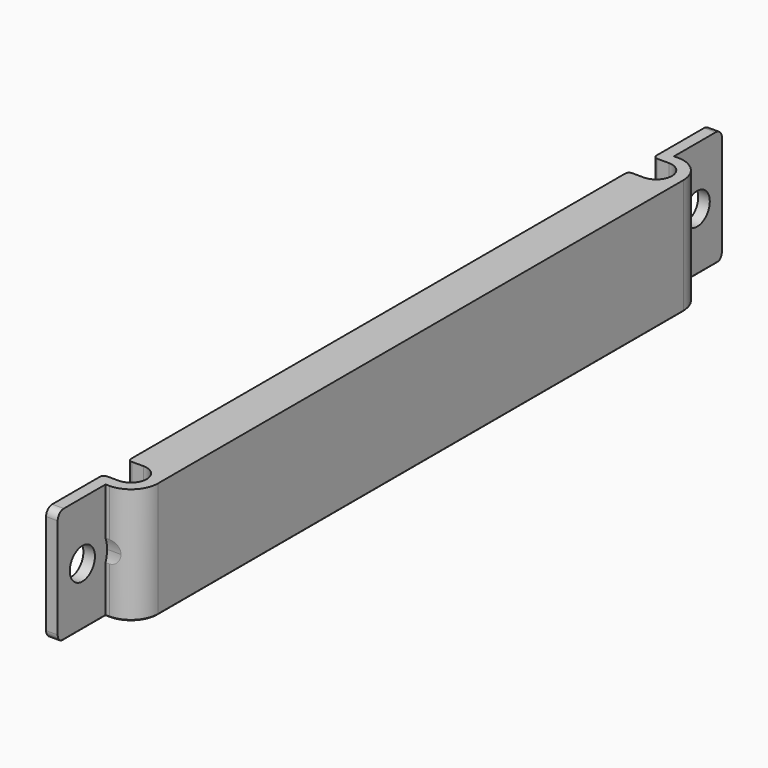
from build123d import *

# Parameters (mm, degrees)
F1_DEPTH     = 15
F2_R         = 1
F3_R         = 4.075
F4_DEPTH     = 3
F3_R_2       = 8
F5_DEPTH     = 8.001
F6_R         = 2
F7_T1_DEPTH  = 16.5429652699
F7_T3_DEPTH  = 3
F7_T5_DEPTH  = 170
F7_T7_DEPTH  = 159.9
F7_T9_DEPTH  = 16.5429652699
F7_T12_ANGLE = 90
F7_T16_DEPTH = 15.2358860169
F7_T21_DEPTH = 1.642920747
F7_T24_ANGLE = 180
F7_T26_ANGLE = 90
F7_T28_ANGLE = 90
F7_T30_ANGLE = 90
F7_T34_DEPTH = 1.642920747
F7_T37_ANGLE = 90
F7_T41_DEPTH = 15.2358860169
F7_T44_ANGLE = 180
F7_T46_ANGLE = 90


# Not quite as in the source:
# - a fillet or chamfer that OpenCascade refuses, or shapes differently, is made with other operations: its cross-section is extruded or revolved along the edge and cut away or added


with BuildPart() as f1:
    # F0 (on Top) → F1 (new body, symmetric)
    with BuildSketch(Plane.XY):
        with BuildLine():
            Line((-4, 89.05), (0, 89.05))
            ThreePointArc((0, 89.05), (4.05, 85), (0, 80.95))
            Line((0, 80.95), (-4, 80.95))
            Line((-4, 80.95), (-4, 0))
            Line((-4, 0), (-4, -80.95))
            Line((-4, -80.95), (0, -80.95))
            ThreePointArc((0, -80.95), (4.05, -85), (0, -89.05))
            Line((0, -89.05), (-4, -89.05))
            Line((-4, -89.05), (-4, -107.5))
            Line((-4, -107.5), (-1, -107.5))
            Line((-1, -107.5), (-1, -92))
            Line((-1, -92), (0, -92))
            ThreePointArc((0, -92), (4.9497474683, -89.9497474683), (7, -85))
            Line((7, -85), (7, 0))
            Line((7, 0), (7, 85))
            ThreePointArc((7, 85), (4.9497474683, 89.9497474683), (0, 92))
            Line((0, 92), (-1, 92))
            Line((-1, 92), (-1, 107.5))
            Line((-1, 107.5), (-4, 107.5))
            Line((-4, 107.5), (-4, 89.05))
        make_face()
    extrude(amount=F1_DEPTH, both=True)

    # F2
    f2_edges = [f1.edges().sort_by_distance(p)[0] for p in [
        (-4, 89.05, 0),
        (-4, 80.95, 0),
        (-4, -89.05, 0),
        (-4, -80.95, 0),
    ]]
    fillet(f2_edges, radius=F2_R)

    # F3 (on face) → F4 (cut, through all)
    with BuildSketch(Plane.YZ.offset(-1)):
        with Locations((99.5, 0)):
            Circle(F3_R)
        with Locations((-99.5, 0)):
            Circle(F3_R)
    extrude(amount=-F4_DEPTH, mode=Mode.SUBTRACT)

    # F3 (on face) → F5 (cut, through all)
    with BuildSketch(Plane.YZ.offset(-1)):
        with Locations((99.5, 0)):
            Circle(F3_R_2)
        with Locations((99.5, 0)):
            Circle(F3_R, mode=Mode.SUBTRACT)
        with BuildLine():
            ThreePointArc((-92, -2.7838821814), (-91.625992126, -1.4142135624), (-91.5, 0))
            ThreePointArc((-91.5, 0), (-91.625992126, 1.4142135624), (-92, 2.7838821814))
            Line((-92, 2.7838821814), (-92, -2.7838821814))
        make_face()
        with BuildLine():
            Line((-92, -2.7838821814), (-92, 2.7838821814))
            ThreePointArc((-92, 2.7838821814), (-100.9142136429, 7.8740078596), (-107.5, -1.636e-07))
            ThreePointArc((-107.5, -1.636e-07), (-100.9142134819, -7.8740078885), (-92, -2.7838821814))
        make_face()
        with Locations((-99.5, 0)):
            Circle(F3_R, mode=Mode.SUBTRACT)
    extrude(amount=F5_DEPTH, mode=Mode.SUBTRACT)

    # F6
    f6_edges = [f1.edges().sort_by_distance(p)[0] for p in [
        (-2.5, 107.5, -15),
        (-2.5, 107.5, 15),
        (-2.5, -107.5, -15),
        (-2.5, -107.5, 15),
    ]]
    fillet(f6_edges, radius=F6_R)

    # F7: chamfer of 0.25 on 22 edges, made by hand

    # F7_s2 → F7_t1 (cut)
    with BuildSketch(Plane.XZ.offset(-106.5929652699)):
        Polygon((-3.75, -15), (-4, -14.75), (-4, -15), align=None)
    extrude(amount=F7_T1_DEPTH, mode=Mode.SUBTRACT)

    # F7_s4 → F7_t3 (cut)
    with BuildSketch(Plane.YZ.offset(-3)):
        Polygon((89.3, -15), (89.05, -14.75), (89.05, -15), align=None)
        Polygon((80.7, -15), (80.95, -14.75), (80.95, -15), align=None)
        Polygon((-80.7, -15), (-80.95, -14.75), (-80.95, -15), align=None)
        Polygon((-89.3, -15), (-89.05, -14.75), (-89.05, -15), align=None)
    extrude(amount=F7_T3_DEPTH, mode=Mode.SUBTRACT)

    # F7_s6 → F7_t5 (cut)
    with BuildSketch(Plane.XZ.offset(-85)):
        Polygon((6.75, -15), (7, -14.75), (7, -15), align=None)
    extrude(amount=F7_T5_DEPTH, mode=Mode.SUBTRACT)

    # F7_s8 → F7_t7 (cut)
    with BuildSketch(Plane.XZ.offset(-79.95)):
        Polygon((-3.75, -15), (-4, -14.75), (-4, -15), align=None)
    extrude(amount=F7_T7_DEPTH, mode=Mode.SUBTRACT)

    # F7_s10 → F7_t9 (cut)
    with BuildSketch(Plane.XZ.offset(90.05)):
        Polygon((-4, -14.75), (-3.75, -15), (-4, -15), align=None)
    extrude(amount=F7_T9_DEPTH, mode=Mode.SUBTRACT)

    # F7_s11 → F7_t12 (revolve, cut)
    with BuildSketch(Plane.YZ.offset(-3)):
        Polygon((89.3, -15), (89.05, -14.75), (89.05, -15), align=None)
    revolve(axis=Axis((-3, 90.05, -15), (0, 0, -1)), revolution_arc=F7_T12_ANGLE, mode=Mode.SUBTRACT)


with BuildPart() as f7_tool14:
    # F7_s15 → F7_t16 (new body)
    with BuildSketch(Plane.XZ.offset(-91.357079253)):
        Polygon((-1.25, -15), (-1, -14.75), (-1, -15), align=None)
    extrude(amount=-F7_T16_DEPTH)

    split(bisect_by=Plane(origin=(0, 53.375, -53.375), x_dir=(1, 0, 0), z_dir=(0, 0.7071067812, -0.7071067812)), keep=Keep.TOP)


with BuildPart() as f1_1:
    add(f1.part)

    # F7_t13: cut F7_tool14
    add(f7_tool14.part, mode=Mode.SUBTRACT)


with BuildPart() as f7_tool19:
    # F7_s20 → F7_t21 (new body)
    with BuildSketch(Plane.YZ):
        Polygon((91.75, -15), (92, -14.75), (92, -15), align=None)
    extrude(amount=-F7_T21_DEPTH)

    split(bisect_by=Plane(origin=(6.875, 0, -6.875), x_dir=(0, 1, 0), z_dir=(0.7071067812, 0, -0.7071067812)), keep=Keep.TOP)


with BuildPart() as f1_2:
    add(f1_1.part)

    # F7_t18: cut F7_tool19
    add(f7_tool19.part, mode=Mode.SUBTRACT)

    # F7_s23 → F7_t24 (revolve, cut)
    with BuildSketch(Plane.YZ):
        Polygon((89.3, -15), (89.05, -14.75), (89.05, -15), align=None)
    revolve(axis=Axis((0, 85, -15), (0, 0, -1)), revolution_arc=F7_T24_ANGLE, mode=Mode.SUBTRACT)

    # F7_s25 → F7_t26 (revolve, cut)
    with BuildSketch(Plane.XZ.offset(-85)):
        Polygon((6.75, -15), (7, -14.75), (7, -15), align=None)
    revolve(axis=Axis((0, 85, -15), (0, 0, 1)), revolution_arc=F7_T26_ANGLE, mode=Mode.SUBTRACT)

    # F7_s27 → F7_t28 (revolve, cut)
    with BuildSketch(Plane.XZ.offset(-79.95)):
        Polygon((-3.75, -15), (-4, -14.75), (-4, -15), align=None)
    revolve(axis=Axis((-3, 79.95, -15), (0, 0, -1)), revolution_arc=F7_T28_ANGLE, mode=Mode.SUBTRACT)

    # F7_s29 → F7_t30 (revolve, cut)
    with BuildSketch(Plane.YZ):
        Polygon((-91.75, -15), (-92, -14.75), (-92, -15), align=None)
    revolve(axis=Axis((0, -85, -15), (0, 0, 1)), revolution_arc=F7_T30_ANGLE, mode=Mode.SUBTRACT)


with BuildPart() as f7_tool32:
    # F7_s33 → F7_t34 (new body)
    with BuildSketch(Plane.YZ.offset(-1.642920747)):
        Polygon((-91.75, -15), (-92, -14.75), (-92, -15), align=None)
    extrude(amount=F7_T34_DEPTH)

    split(bisect_by=Plane(origin=(6.875, 0, -6.875), x_dir=(0, 1, 0), z_dir=(0.7071067812, 0, -0.7071067812)), keep=Keep.TOP)


with BuildPart() as f1_3:
    add(f1_2.part)

    # F7_t31: cut F7_tool32
    add(f7_tool32.part, mode=Mode.SUBTRACT)

    # F7_s36 → F7_t37 (revolve, cut)
    with BuildSketch(Plane.YZ.offset(-3)):
        Polygon((-80.7, -15), (-80.95, -14.75), (-80.95, -15), align=None)
    revolve(axis=Axis((-3, -79.95, -15), (0, 0, -1)), revolution_arc=F7_T37_ANGLE, mode=Mode.SUBTRACT)


with BuildPart() as f7_tool39:
    # F7_s40 → F7_t41 (new body)
    with BuildSketch(Plane.XZ.offset(106.5929652699)):
        Polygon((-1.25, -15), (-1, -14.75), (-1, -15), align=None)
    extrude(amount=-F7_T41_DEPTH)

    split(bisect_by=Plane(origin=(0, -53.375, -53.375), x_dir=(1, 0, 0), z_dir=(0, -0.7071067812, -0.7071067812)), keep=Keep.TOP)


with BuildPart() as f1_4:
    add(f1_3.part)

    # F7_t38: cut F7_tool39
    add(f7_tool39.part, mode=Mode.SUBTRACT)

    # F7_s43 → F7_t44 (revolve, cut)
    with BuildSketch(Plane.YZ):
        Polygon((-80.7, -15), (-80.95, -14.75), (-80.95, -15), align=None)
    revolve(axis=Axis((0, -85, -15), (0, 0, -1)), revolution_arc=F7_T44_ANGLE, mode=Mode.SUBTRACT)

    # F7_s45 → F7_t46 (revolve, cut)
    with BuildSketch(Plane.XZ.offset(90.05)):
        Polygon((-3.75, -15), (-4, -14.75), (-4, -15), align=None)
    revolve(axis=Axis((-3, -90.05, -15), (0, 0, -1)), revolution_arc=F7_T46_ANGLE, mode=Mode.SUBTRACT)


solid = f1_4.part
